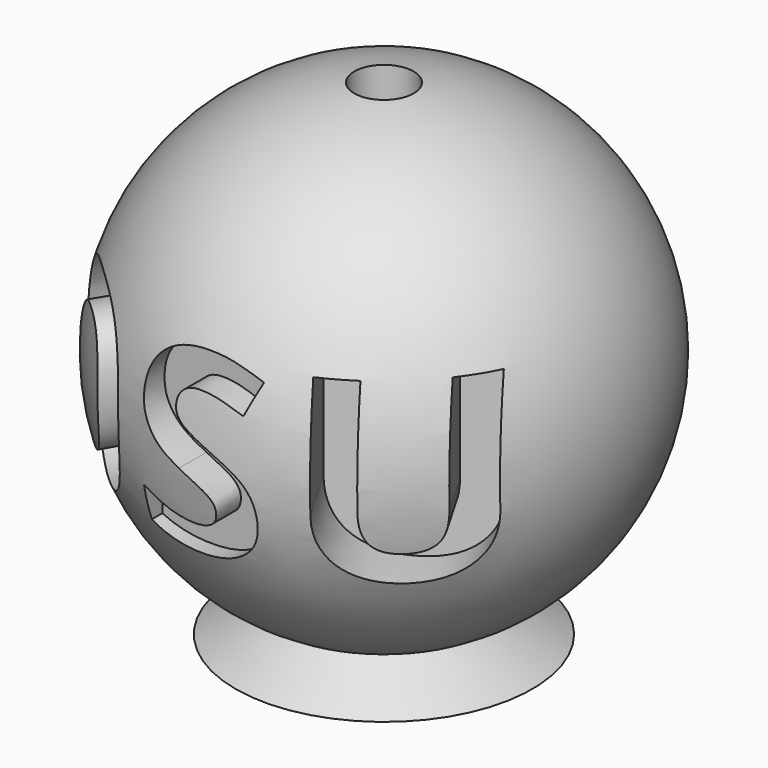
from build123d import *

# Parameters (mm, degrees)
F2_R          = 3.175
F3_DEPTH      = 50.8
F8_TEXT_SIZE  = 26.4583333333
F11_DEPTH     = 10.16
F9_TEXT_SIZE  = 26.4583333333
F12_DEPTH     = 15.24
F10_TEXT_SIZE = 26.4583333333
F13_DEPTH     = 15.24
F16_R         = 9.525
F17_DEPTH     = 38.1


# Not quite as in the source:
# - Text() gives the source's letters only with a copy of the font that has no kerning and outlines rounded to 1/6400 em; it was checked with that copy


with BuildPart() as f1:
    # F0 (on Front) → F1 (revolve)
    with BuildSketch(Plane.XZ):
        with BuildLine():
            Line((0, -25.4), (0, 25.4))
            ThreePointArc((0, 25.4), (-25.4, 0), (0, -25.4))
        make_face()
    revolve(axis=Axis((0, 0, 0), (0, 0, -1)))

    # F2 (on Top) → F3 (cut, symmetric)
    with BuildSketch(Plane.XY):
        Circle(F2_R)
    extrude(amount=F3_DEPTH, both=True, mode=Mode.SUBTRACT)

    # F8 (on offset) → F11 (cut)
    with BuildSketch(Plane.XZ.offset(31.75)):
        with Locations((-7.6212402344, -9.525)):
            Text('S', F8_TEXT_SIZE, font='Open Sans', font_style=FontStyle.BOLD, text_align=(TextAlign.LEFT, TextAlign.BOTTOM))
    extrude(amount=-F11_DEPTH, mode=Mode.SUBTRACT)

    # F9 (on face) → F12 (cut)
    with BuildSketch(Plane(origin=(-16.4977839421, -28.575, 0), x_dir=(-0.8660254038, 0.5, 0), z_dir=(0.5, 0.8660254038, 0))):
        with Locations((-4.992239809, -9.9285113379)):
            Text('O', F9_TEXT_SIZE, font='Open Sans', font_style=FontStyle.BOLD, text_align=(TextAlign.LEFT, TextAlign.BOTTOM))
    extrude(amount=F12_DEPTH, mode=Mode.SUBTRACT)

    # F10 (on face) → F13 (cut)
    with BuildSketch(Plane(origin=(16.4977839421, -28.575, 0), x_dir=(-0.8660254038, -0.5, 0), z_dir=(-0.5, 0.8660254038, 0))):
        with Locations((-15.3599997865, -9.525)):
            Text('U', F10_TEXT_SIZE, font='Open Sans', font_style=FontStyle.BOLD, text_align=(TextAlign.LEFT, TextAlign.BOTTOM))
    extrude(amount=F13_DEPTH, mode=Mode.SUBTRACT)

    # F16 (on offset) → F17 (cut)
    with BuildSketch(Plane.XY.offset(-25.4)):
        Circle(F16_R)
    extrude(amount=F17_DEPTH, mode=Mode.SUBTRACT)

    # F18 (on Front) → F19 (revolve)
    with BuildSketch(Plane.XZ):
        Polygon((-9.525, -23.5464301965), (-10.0812907232, -23.240218454), (-15.875, -26.7214301965), (-9.525, -26.7214301965), align=None)
    revolve(axis=Axis((0, 0, 19.05), (0, 0, 1)))


solid = f1.part
